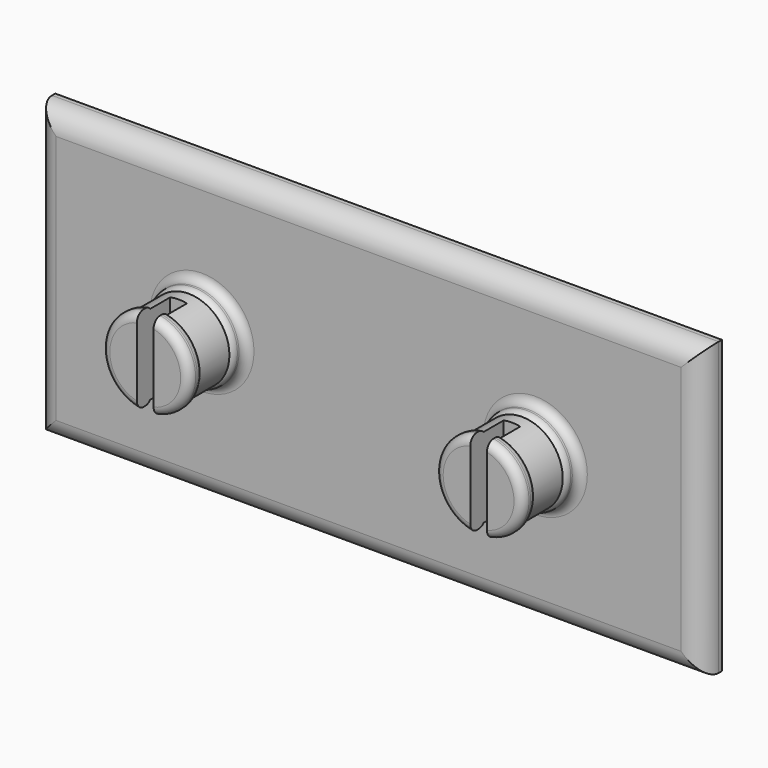
from build123d import *

# Parameters (mm, degrees)
F0_W      = 80
F0_H      = 35
F1_DEPTH  = 3
F2_R      = 5.25
F3_DEPTH  = 2
F4_R      = 4.9
F5_DEPTH  = 4.5
F6_R      = 5.25
F7_DEPTH  = 2
F9_W      = 2
F9_H      = 15
F10_DEPTH = 5
F11_R     = 2.5


# Not quite as in the source:
# - a fillet or chamfer that OpenCascade refuses, or shapes differently, is made with other operations: its cross-section is extruded or revolved along the edge and cut away or added


with BuildPart() as f1:
    # F0 (on Front) → F1 (new body)
    with BuildSketch(Plane.XZ):
        Rectangle(F0_W, F0_H)
    extrude(amount=F1_DEPTH)

    # F2 (on face) → F3 (join)
    with BuildSketch(Plane.XZ.offset(3)):
        with Locations((-20, 0)):
            Circle(F2_R)
        with Locations((20, 0)):
            Circle(F2_R)
    extrude(amount=F3_DEPTH)

    # F4 (on face) → F5 (join)
    with BuildSketch(Plane.XZ.offset(5)):
        with Locations((-20, 0)):
            Circle(F4_R)
        with Locations((20, 0)):
            Circle(F4_R)
    extrude(amount=F5_DEPTH)

    # F6 (on face) → F7 (join)
    with BuildSketch(Plane.XZ.offset(9.5)):
        with Locations((-20, 0)):
            Circle(F6_R)
        with Locations((20, 0)):
            Circle(F6_R)
    extrude(amount=F7_DEPTH)

    # F8: fillet of radius 1 on 8 edges, made by hand

    # F8_s1 → F8_t2 (revolve)
    with BuildSketch(Plane.XY):
        with BuildLine():
            ThreePointArc((-14.75, -4), (-14.4571067812, -3.2928932188), (-13.75, -3))
            Line((-13.75, -3), (-14.75, -3))
            Line((-14.75, -3), (-14.75, -4))
        make_face()
    revolve(axis=Axis((-20, -3, 0), (0, -1, 0)))

    # F8_s3 → F8_t4 (revolve)
    with BuildSketch(Plane.XY):
        with BuildLine():
            ThreePointArc((26.25, -3), (25.5428932188, -3.2928932188), (25.25, -4))
            Line((25.25, -4), (25.25, -3))
            Line((25.25, -3), (26.25, -3))
        make_face()
    revolve(axis=Axis((20, -3, 0), (0, -1, 0)))

    # F8_s5 → F8_t6 (revolve, cut)
    with BuildSketch(Plane.XY):
        with BuildLine():
            ThreePointArc((-14.75, -10.2599342077), (-14.8417048938, -9.8416041944), (-15.1, -9.5))
            Line((-15.1, -9.5), (-14.75, -9.5))
            Line((-14.75, -9.5), (-14.75, -10.2599342077))
        make_face()
    revolve(axis=Axis((-20, -9.5, 0), (0, -1, 0)), mode=Mode.SUBTRACT)

    # F8_s7 → F8_t8 (revolve, cut)
    with BuildSketch(Plane.XY):
        with BuildLine():
            ThreePointArc((-14.75, -10.5), (-15.0428932188, -11.2071067812), (-15.75, -11.5))
            Line((-15.75, -11.5), (-14.75, -11.5))
            Line((-14.75, -11.5), (-14.75, -10.5))
        make_face()
    revolve(axis=Axis((-20, -11.5, 0), (0, -1, 0)), mode=Mode.SUBTRACT)

    # F8_s9 → F8_t10 (revolve, cut)
    with BuildSketch(Plane.XY):
        with BuildLine():
            ThreePointArc((-15.1, -5), (-14.8417048938, -4.6583958056), (-14.75, -4.2400657923))
            Line((-14.75, -4.2400657923), (-14.75, -5))
            Line((-14.75, -5), (-15.1, -5))
        make_face()
    revolve(axis=Axis((-20, -5, 0), (0, -1, 0)), mode=Mode.SUBTRACT)

    # F8_s11 → F8_t12 (revolve, cut)
    with BuildSketch(Plane.XY):
        with BuildLine():
            ThreePointArc((25.25, -4.2400657923), (25.1582951062, -4.6583958056), (24.9, -5))
            Line((24.9, -5), (25.25, -5))
            Line((25.25, -5), (25.25, -4.2400657923))
        make_face()
    revolve(axis=Axis((20, -5, 0), (0, -1, 0)), mode=Mode.SUBTRACT)

    # F8_s13 → F8_t14 (revolve, cut)
    with BuildSketch(Plane.XY):
        with BuildLine():
            ThreePointArc((24.9, -9.5), (25.1582951062, -9.8416041944), (25.25, -10.2599342077))
            Line((25.25, -10.2599342077), (25.25, -9.5))
            Line((25.25, -9.5), (24.9, -9.5))
        make_face()
    revolve(axis=Axis((20, -9.5, 0), (0, -1, 0)), mode=Mode.SUBTRACT)

    # F8_s15 → F8_t16 (revolve, cut)
    with BuildSketch(Plane.XY):
        with BuildLine():
            ThreePointArc((25.25, -10.5), (24.9571067812, -11.2071067812), (24.25, -11.5))
            Line((24.25, -11.5), (25.25, -11.5))
            Line((25.25, -11.5), (25.25, -10.5))
        make_face()
    revolve(axis=Axis((20, -11.5, 0), (0, -1, 0)), mode=Mode.SUBTRACT)

    # F9 (on face) → F10 (cut)
    with BuildSketch(Plane.XZ.offset(11.5)):
        with Locations((-20, 0)):
            Rectangle(F9_W, F9_H)
        with Locations((20, 0)):
            Rectangle(F9_W, F9_H)
    extrude(amount=-F10_DEPTH, mode=Mode.SUBTRACT)

    # F11
    f11_edges = [f1.edges().sort_by_distance(p)[0] for p in [
        (-40, -3, 0),
        (0, -3, 17.5),
        (40, -3, 0),
        (0, -3, -17.5),
    ]]
    fillet(f11_edges, radius=F11_R)


solid = f1.part
